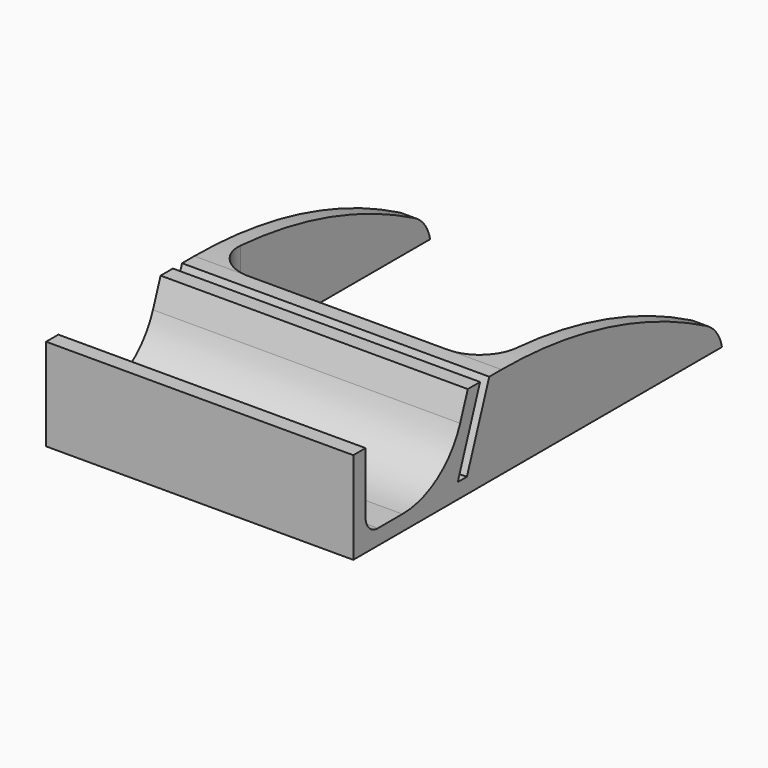
from build123d import *

# Parameters (mm, degrees)
F1_DEPTH    = 40
F2_R        = 10
F3_R        = 2
F4_W        = 36
F4_H        = 35.8704487759
F5_DEPTH    = 25
F6_R        = 5
F7_T1_DEPTH = 16.4561700335
F7_T3_DEPTH = 16.4561700335


# Not quite as in the source:
# - a fillet or chamfer that OpenCascade refuses, or shapes differently, is made with other operations: its cross-section is extruded or revolved along the edge and cut away or added


with BuildPart() as f1:
    # F0 (on Right) → F1 (new body)
    with BuildSketch(Plane.YZ):
        Polygon((13, 0), (0, 0), (0, 10), (-2, 10), (-2, -2), (58, -2), (58, 0), (22.1295512241, 0), (22.1295512241, 10), (20.1295512241, 10), (16.4898488815, 0), (15, 0), (18.6397023427, 10), (16.6397023427, 10), align=None)
        with BuildLine():
            Line((22.1295512241, 0), (58, 0))
            ThreePointArc((58, 0), (40.7486885255, 7.4532263127), (22.1295512241, 10))
            Line((22.1295512241, 10), (22.1295512241, 0))
        make_face()
    extrude(amount=F1_DEPTH)

    # F2
    f2_edges = [f1.edges().sort_by_distance(p)[0] for p in [
        (20, 13, 0),
    ]]
    fillet(f2_edges, radius=F2_R)

    # F3
    f3_edges = [f1.edges().sort_by_distance(p)[0] for p in [
        (20, 0, 0),
    ]]
    fillet(f3_edges, radius=F3_R)

    # F4 (on face) → F5 (cut)
    with BuildSketch(Plane.XY.offset(10)):
        with Locations((20, 40.0647756121)):
            Rectangle(F4_W, F4_H)
    extrude(amount=-F5_DEPTH, mode=Mode.SUBTRACT)

    # F6
    f6_edges = [f1.edges().sort_by_distance(p)[0] for p in [
        (2, 22.129551, 4),
        (38, 22.129551, 4),
    ]]
    fillet(f6_edges, radius=F6_R)

    # F7: fillet of radius 5 on 2 edges, made by hand

    # F7_s2 → F7_t1 (cut)
    with BuildSketch(Plane.YZ.offset(-7.2280850168)):
        with BuildLine():
            ThreePointArc((58, -2), (57.132526229, 0.0019440058), (55.4951149029, 1.4438783647))
            ThreePointArc((55.4951149029, 1.4438783647), (56.7550844524, 0.7349972576), (58, 0))
            Line((58, 0), (58, -2))
        make_face()
    extrude(amount=F7_T1_DEPTH, mode=Mode.SUBTRACT)

    # F7_s4 → F7_t3 (cut)
    with BuildSketch(Plane.YZ.offset(30.7719149832)):
        with BuildLine():
            ThreePointArc((58, -2), (57.132526229, 0.0019440058), (55.4951149029, 1.4438783647))
            ThreePointArc((55.4951149029, 1.4438783647), (56.7550844524, 0.7349972576), (58, 0))
            Line((58, 0), (58, -2))
        make_face()
    extrude(amount=F7_T3_DEPTH, mode=Mode.SUBTRACT)


solid = f1.part
